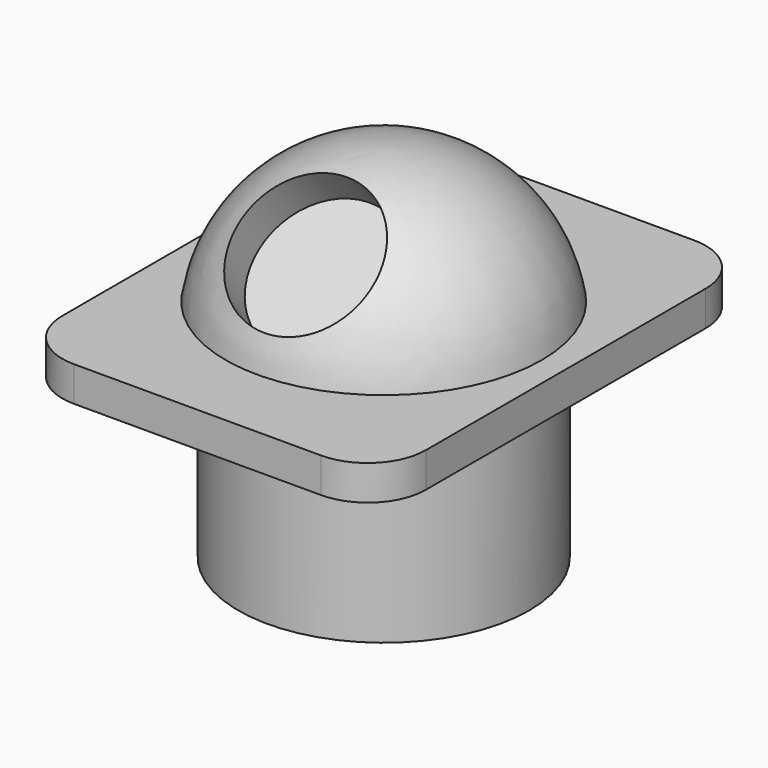
from build123d import *

# Parameters (mm, degrees)
F0_R      = 10
F1_DEPTH  = 13
F2_W      = 25
F2_H      = 32.05
F2_R      = 10
F3_DEPTH  = 2.4
F4_R      = 4
F9_R      = 4.8243357568
F10_DEPTH = 3.9818781354


with BuildPart() as f1:
    # F0 (on Top) → F1 (new body)
    with BuildSketch(Plane.XY):
        Circle(F0_R)
    extrude(amount=-F1_DEPTH)

    # F2 (on face) → F3 (join)
    with BuildSketch(Plane.XY):
        with Locations((0, 0.025)):
            Rectangle(F2_W, F2_H)
        Circle(F2_R, mode=Mode.SUBTRACT)
        Circle(F2_R)
    extrude(amount=F3_DEPTH)

    # F4
    f4_edges = [f1.edges().sort_by_distance(p)[0] for p in [
        (-12.5, -16, 1.2),
        (12.5, -16, 1.2),
        (12.5, 16.05, 1.2),
        (-12.5, 16.05, 1.2),
    ]]
    fillet(f4_edges, radius=F4_R)


with BuildPart() as f6:
    # F5 (on Front) → F6 (revolve)
    with BuildSketch(Plane.XZ):
        with BuildLine():
            Line((0, 2.4442088325), (10.8725447208, 2.4442088325))
            ThreePointArc((10.8725447208, 2.4442088325), (7.1545871503, 9.0910971974), (0, 11.7018856108))
            Line((0, 11.7018856108), (0, 2.4442088325))
        make_face()
    revolve(axis=Axis((0, 0, 8.3999085473), (0, 0, 1)))

    # F9 (on face) → F10 (cut, through all)
    with BuildSketch(Plane(origin=(0, -4.8739186494, 5.8085100605), x_dir=(1, 0, 0), z_dir=(0, -0.6427876097, 0.7660444431))):
        Circle(F9_R)
    extrude(amount=F10_DEPTH, mode=Mode.SUBTRACT)


solid = Compound([f1.part, f6.part])
